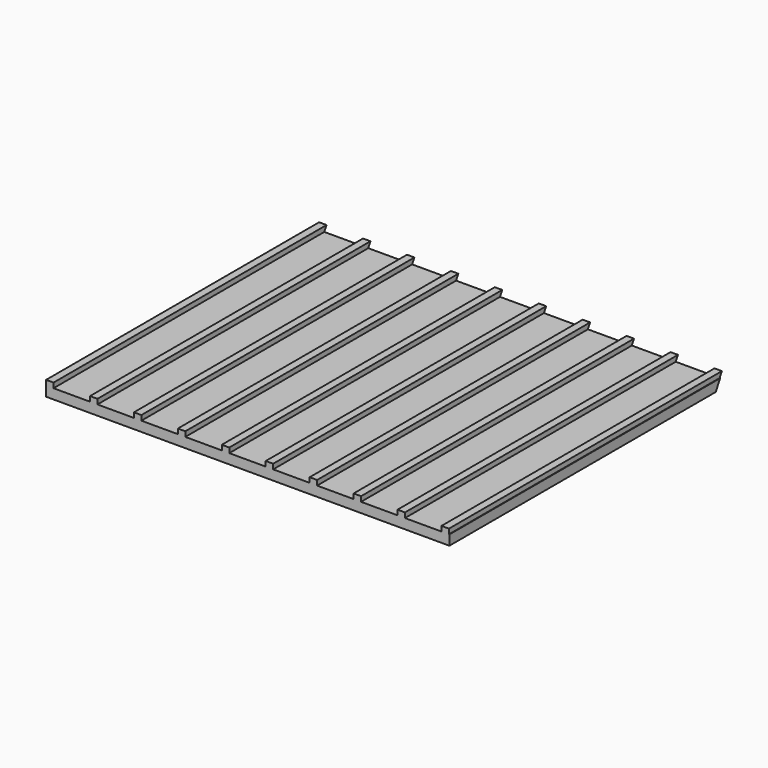
from build123d import *

# Parameters (mm, degrees)
F0_W     = 82.55
F0_H     = 69.85
F1_DEPTH = 2.032
F2_W     = 1.524
F2_H     = 69.85
F3_DEPTH = 1.016
F5_DEPTH = 88.8746


with BuildPart() as f1:
    # F0 (on Top) → F1 (new body)
    with BuildSketch(Plane.XY):
        with Locations((-16.0199867169, 0.6959252059)):
            Rectangle(F0_W, F0_H)
    extrude(amount=F1_DEPTH)

    # F2 (on face) → F3 (join)
    with BuildSketch(Plane.XY.offset(2.032)):
        with Locations((-56.5329867169, 0.6959252059)):
            Rectangle(F2_W, F2_H)
        with Locations((-47.5413867169, 0.6959252059)):
            Rectangle(F2_W, F2_H)
        with Locations((-38.5497867169, 0.6959252059)):
            Rectangle(F2_W, F2_H)
        with Locations((-29.5581867169, 0.6959252059)):
            Rectangle(F2_W, F2_H)
        with Locations((-20.5665867169, 0.6959252059)):
            Rectangle(F2_W, F2_H)
        with Locations((-11.5749867169, 0.6959252059)):
            Rectangle(F2_W, F2_H)
        with Locations((-2.5833867169, 0.6959252059)):
            Rectangle(F2_W, F2_H)
        with Locations((6.4082132831, 0.6959252059)):
            Rectangle(F2_W, F2_H)
        with Locations((15.3998132831, 0.6959252059)):
            Rectangle(F2_W, F2_H)
        with Locations((24.3914132831, 0.6959252059)):
            Rectangle(F2_W, F2_H)
    extrude(amount=F3_DEPTH)

    # F4 (on face) → F5 (cut)
    with BuildSketch(Plane.YZ.offset(25.2550132831)):
        Polygon((33.9077030866, 0), (33.703327179, -0.3639321658), (35.670414567, -0.3639321658), (35.670414567, 3.138860222), (35.048827404, 2.032), (35.6209252059, 2.032), (35.6209252059, 0), align=None)
        Polygon((35.048827404, 2.032), (33.9077030866, 0), (35.6209252059, 0), (35.6209252059, 2.032), align=None)
    extrude(amount=-F5_DEPTH, mode=Mode.SUBTRACT)


solid = f1.part
